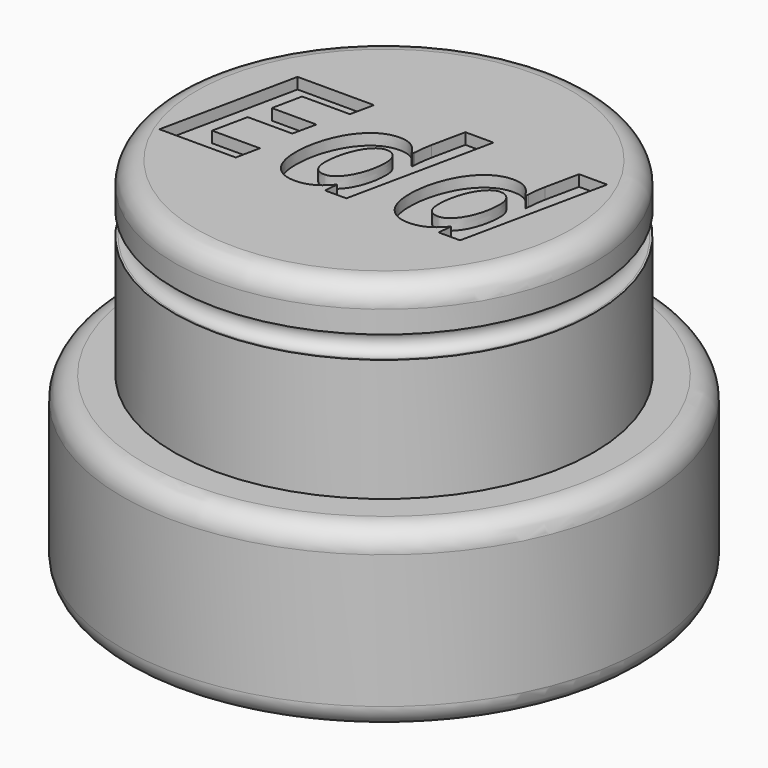
from build123d import *

# Parameters (mm, degrees)
F0_R         = 23.5
F0_R_2       = 18.85
F1_DEPTH     = 16
F2_DEPTH     = 33
F3_R         = 2
F6_TEXT_SIZE = 17.1925690805
F7_DEPTH     = 1


# Not quite as in the source:
# - Text() gives the source's letters only with a copy of the font that has no kerning and outlines rounded to 1/6400 em; it was checked with that copy


with BuildPart() as f1:
    # F0 (on Top) → F1 (new body)
    with BuildSketch(Plane.XY):
        Circle(F0_R)
        Circle(F0_R_2, mode=Mode.SUBTRACT)
    extrude(amount=F1_DEPTH)

    # F0 (on Top) → F2 (join)
    with BuildSketch(Plane.XY):
        Circle(F0_R_2)
    extrude(amount=F2_DEPTH)

    # F3
    f3_edges = [f1.edges().sort_by_distance(p)[0] for p in [
        (-18.85, 0, 33),
        (-23.5, 0, 16),
        (-23.5, 0, 0),
    ]]
    fillet(f3_edges, radius=F3_R)

    # F4 (on Front) → F5 (revolve, cut)
    with BuildSketch(Plane.XZ):
        with BuildLine():
            ThreePointArc((19.1321484745, 27.1126012729), (19.525839484, 27.4808674113), (19.6711457638, 28))
            ThreePointArc((19.6711457638, 28), (19.4696919186, 28.6019335833), (18.9464976863, 28.9613434968))
            ThreePointArc((18.9464976863, 28.9613434968), (18.7991912387, 28.9917682977), (18.6489877804, 28.9997544817))
            ThreePointArc((18.6489877804, 28.9997544817), (17.6712071453, 27.9889203282), (18.6711457638, 27))
            ThreePointArc((18.6711457638, 27), (18.9084233154, 27.0285581008), (19.1321484745, 27.1126012729))
        make_face()
        with BuildLine():
            ThreePointArc((18.6489877804, 28.9997544817), (18.7991912387, 28.9917682977), (18.9464976863, 28.9613434968))
            Line((18.9464976863, 28.9613434968), (18.945500715, 29.0063262239))
            Line((18.945500715, 29.0063262239), (18.6489877804, 28.9997544817))
        make_face()
        with BuildLine():
            Line((19.1321484745, 27), (19.1321484745, 27.1126012729))
            ThreePointArc((19.1321484745, 27.1126012729), (18.9084233154, 27.0285581008), (18.6711457638, 27))
            Line((18.6711457638, 27), (19.1321484745, 27))
        make_face()
    revolve(axis=Axis((0, 0, 18.8947152346), (0, 0, 1)), mode=Mode.SUBTRACT)

    # F6 (on face) → F7 (cut)
    with BuildSketch(Plane.XY.offset(33)):
        with Locations((-15.6721012524, -6.189324869)):
            Text('Edd', F6_TEXT_SIZE, font='Open Sans', font_style=FontStyle.BOLDITALIC, text_align=(TextAlign.LEFT, TextAlign.BOTTOM))
    extrude(amount=-F7_DEPTH, mode=Mode.SUBTRACT)


solid = f1.part
